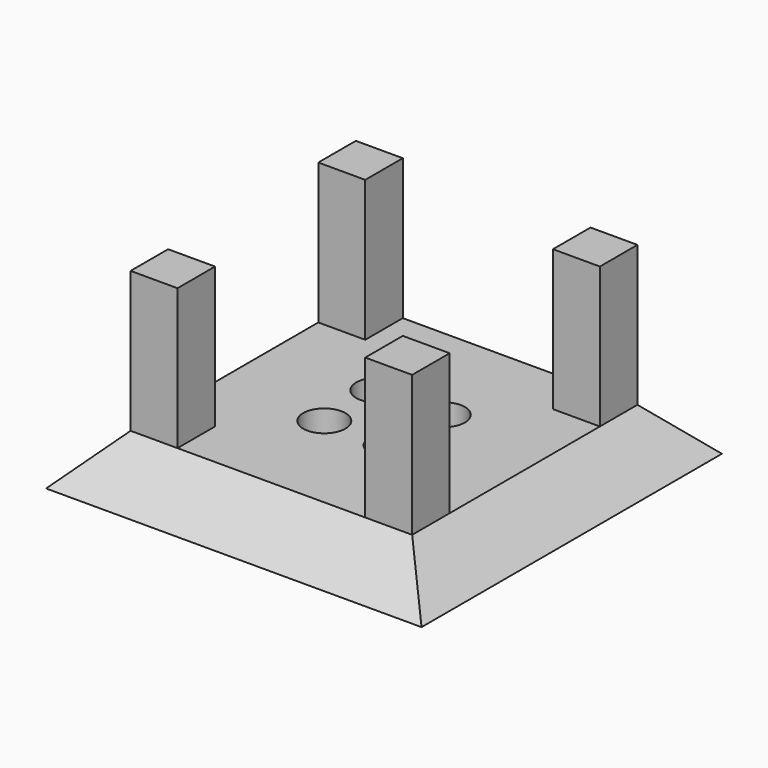
from build123d import *

# Parameters (mm, degrees)
F0_W     = 80
F0_H     = 80
F1_DEPTH = 10
F2_SIZE2 = 9.99999
F2_SIZE  = 9.99999
F3_W     = 10
F3_H     = 10
F4_DEPTH = 30
F6_DEPTH = 8


# Not quite as in the source:
# - a fillet or chamfer is up to 0.001 mm smaller than in the source, because OpenCascade refuses the exact size


with BuildPart() as f1:
    # F0 (on Top) → F1 (new body)
    with BuildSketch(Plane.XY):
        Rectangle(F0_W, F0_H)
    extrude(amount=F1_DEPTH)

    # F2 (size 10 and 10 in the source; OpenCascade refuses exactly that, so slightly less here)
    f2_edges = [f1.edges().sort_by_distance(p)[0] for p in [
        (0, 40, 10),
        (-40, 0, 10),
        (0, -40, 10),
        (40, 0, 10),
    ]]
    chamfer(f2_edges, length=F2_SIZE, length2=F2_SIZE2)

    # F3 (on face) → F4 (join)
    with BuildSketch(Plane.XY.offset(10)):
        with Locations((-25, 25)):
            Rectangle(F3_W, F3_H)
        with Locations((-25, -25)):
            Rectangle(F3_W, F3_H)
        with Locations((25, 25)):
            Rectangle(F3_W, F3_H)
        with Locations((25, -25)):
            Rectangle(F3_W, F3_H)
    extrude(amount=F4_DEPTH)

    # F5 (on face) → F6 (cut)
    with BuildSketch(Plane.XY.offset(10)):
        with BuildLine():
            Line((-3.8890872965, 3.8890872965), (-10.2530483272, 10.2530483272))
            ThreePointArc((-10.2530483272, 10.2530483272), (-10.2530483272, 3.8890872965), (-3.8890872965, 3.8890872965))
        make_face()
        with BuildLine():
            ThreePointArc((-2.5710678119, 7.0710678119), (-5.3489923662, 11.2285257082), (-10.2530483272, 10.2530483272))
            Line((-10.2530483272, 10.2530483272), (-3.8890872965, 3.8890872965))
            ThreePointArc((-3.8890872965, 3.8890872965), (-2.9136099156, 5.3489923662), (-2.5710678119, 7.0710678119))
        make_face()
        with BuildLine():
            ThreePointArc((10.2530483272, 10.2530483272), (3.8890872965, 10.2530483272), (3.8890872965, 3.8890872965))
            Line((3.8890872965, 3.8890872965), (10.2530483272, 10.2530483272))
        make_face()
        with BuildLine():
            Line((10.2530483272, 10.2530483272), (3.8890872965, 3.8890872965))
            ThreePointArc((3.8890872965, 3.8890872965), (8.7931432575, 2.9136099156), (11.5710678119, 7.0710678119))
            ThreePointArc((11.5710678119, 7.0710678119), (11.2285257082, 8.7931432575), (10.2530483272, 10.2530483272))
        make_face()
        with BuildLine():
            Line((-10.2530483272, -10.2530483272), (-3.8890872965, -3.8890872965))
            ThreePointArc((-3.8890872965, -3.8890872965), (-10.2530483272, -3.8890872965), (-10.2530483272, -10.2530483272))
        make_face()
        with BuildLine():
            ThreePointArc((-2.5710678119, -7.0710678119), (-2.9136099156, -5.3489923662), (-3.8890872965, -3.8890872965))
            Line((-3.8890872965, -3.8890872965), (-10.2530483272, -10.2530483272))
            ThreePointArc((-10.2530483272, -10.2530483272), (-5.3489923662, -11.2285257082), (-2.5710678119, -7.0710678119))
        make_face()
        with BuildLine():
            Line((10.2530483272, -10.2530483272), (3.8890872965, -3.8890872965))
            ThreePointArc((3.8890872965, -3.8890872965), (3.8890872965, -10.2530483272), (10.2530483272, -10.2530483272))
        make_face()
        with BuildLine():
            ThreePointArc((11.5710678119, -7.0710678119), (8.7931432575, -2.9136099156), (3.8890872965, -3.8890872965))
            Line((3.8890872965, -3.8890872965), (10.2530483272, -10.2530483272))
            ThreePointArc((10.2530483272, -10.2530483272), (11.2285257082, -8.7931432575), (11.5710678119, -7.0710678119))
        make_face()
    extrude(amount=-F6_DEPTH, mode=Mode.SUBTRACT)


solid = f1.part
